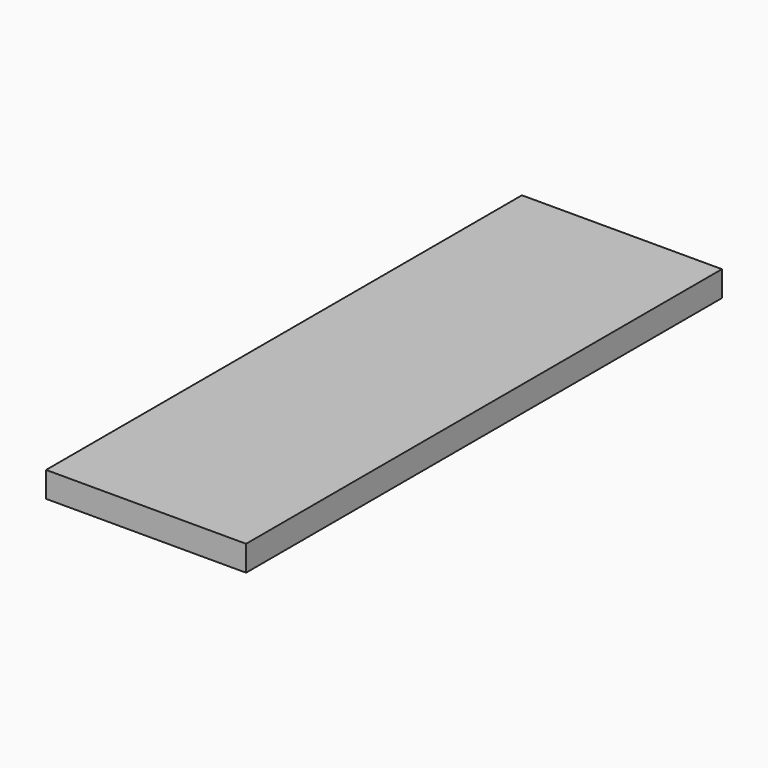
from build123d import *

# Parameters (mm, degrees)
F0_W     = 31.3893184066
F0_H     = 93.3416113257
F1_DEPTH = 4


# Not quite as in the source:
# - the program builds the solid bodies; features that only make, move or delete a surface that nothing else refers to are left out


with BuildPart() as f1:
    # F0 (on Top) → F1 (new body)
    with BuildSketch(Plane.XY):
        with Locations((25.0491015613, 14.7016607225)):
            Rectangle(F0_W, F0_H)
    extrude(amount=F1_DEPTH)


solid = f1.part
